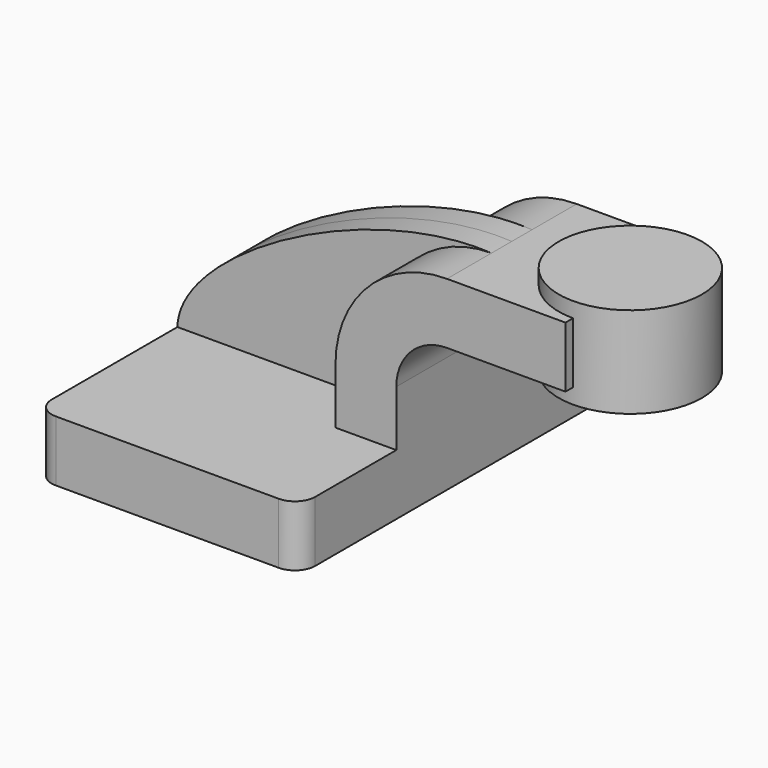
from build123d import *

# Parameters (mm, degrees)
F1_DEPTH = 63.5
F0_W     = 28.3603538342
F0_H     = 19.05
F2_DEPTH = 25.4
F3_DEPTH = 7.9375
F5_R     = 6.35


with BuildPart() as f1:
    # F0 (on Front) → F1 (new body, symmetric)
    with BuildSketch(Plane.XZ):
        Polygon((-41.275, 9.525), (-41.275, -9.525), (41.275, -9.525), (41.275, 9.525), (22.225, 9.525), align=None)
    extrude(amount=F1_DEPTH, both=True)

    # F0 (on Front) → F2 (join, symmetric)
    with BuildSketch(Plane.XZ):
        with BuildLine():
            Line((22.225, 9.525), (41.275, 9.525))
            Line((41.275, 9.525), (41.275, 27.0002))
            ThreePointArc((41.275, 27.0002), (45.9246798487, 38.2255201513), (57.15, 42.8752))
            Line((57.15, 42.8752), (65.9289314961, 42.8752))
            Line((65.9289314961, 42.8752), (65.9289314961, 61.9252))
            Line((65.9289314961, 61.9252), (57.15, 61.9252))
            ThreePointArc((57.15, 61.9252), (32.4542956671, 51.6959043329), (22.225, 27.0002))
            Line((22.225, 27.0002), (22.225, 9.525))
        make_face()
        with Locations((80.1091084132, 52.4002)):
            Rectangle(F0_W, F0_H)
    extrude(amount=F2_DEPTH, both=True)

    # F0 (on Front) → F3 (join, symmetric)
    with BuildSketch(Plane.XZ):
        with BuildLine():
            add(Edge.make_bspline(
                [(-41.275, 9.525), (-40.676958859, 32.2595275939), (17.6535416394, 64.1468688846), (57.15, 61.9252)],
                knots=[0, 0, 0, 0, 111.5045361635, 111.5045361635, 111.5045361635, 111.5045361635], degree=3))
            Line((-41.275, 9.525), (22.225, 9.525))
            Line((22.225, 9.525), (22.225, 27.0002))
            ThreePointArc((22.225, 27.0002), (32.4542956671, 51.6959043329), (57.15, 61.9252))
        make_face()
    extrude(amount=F3_DEPTH, both=True)

    # F5
    f5_edges = [f1.edges().sort_by_distance(p)[0] for p in [
        (41.275, -63.5, 0),
        (-41.275, -63.5, 0),
        (41.275, 63.5, 0),
        (-41.275, 63.5, 0),
    ]]
    fillet(f5_edges, radius=F5_R)


with BuildPart() as f4:
    # F0 (on Front) → F4 (revolve)
    with BuildSketch(Plane.XZ):
        Polygon((94.2892853303, 66.675), (94.2892853303, 61.9252), (94.2892853303, 42.8752), (94.2892853303, 38.1), (116.7289314961, 38.1), (116.7289314961, 66.675), align=None)
    revolve(axis=Axis((94.2892853303, 0, 52.3875), (0, 0, 1)))


solid = Compound([f1.part, f4.part])
